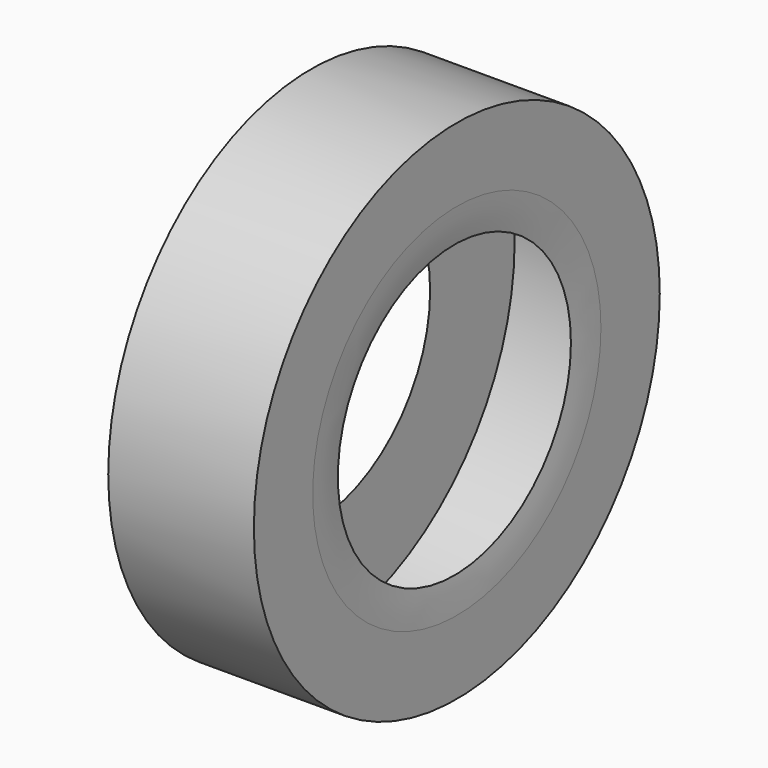
from build123d import *

# Parameters (mm, degrees)
F0_R     = 265.437423464
F0_R_2   = 152.4
F1_DEPTH = 152.4
F2_T     = -2.54


# Not quite as in the source:
# - a fillet or chamfer that OpenCascade refuses, or shapes differently, is made with other operations: its cross-section is extruded or revolved along the edge and cut away or added


with BuildPart() as f1:
    # F0 (on Right) → F1 (new body)
    with BuildSketch(Plane.YZ):
        Circle(F0_R)
        Circle(F0_R_2, mode=Mode.SUBTRACT)
    extrude(amount=F1_DEPTH)

    # F2
    f2_openings = [f1.faces().sort_by_distance(p)[0] for p in [
        (76.2, -152.4, 0),
    ]]
    offset(amount=F2_T, openings=f2_openings)

    # F3: fillet of radius 257.548302834 on 1 edges, made by hand

    # F3_s1 → F3_t2 (revolve, cut)
    with BuildSketch(Plane.XY):
        with BuildLine():
            ThreePointArc((152.4, 188.4817651785), (151.7642152496, 170.3962365824), (149.86, 152.4))
            Line((149.86, 152.4), (152.4, 152.4))
            Line((152.4, 152.4), (152.4, 188.4817651785))
        make_face()
    revolve(axis=Axis((152.4, 0, 0), (1, 0, 0)), mode=Mode.SUBTRACT)

    # F4: fillet of radius 331.1335322151 on 1 edges, made by hand

    # F4_s1 → F4_t2 (revolve, cut)
    with BuildSketch(Plane.XY):
        with BuildLine():
            ThreePointArc((0, 193.3353971967), (0.635610026, 172.828335342), (2.54, 152.4))
            Line((2.54, 152.4), (0, 152.4))
            Line((0, 152.4), (0, 193.3353971967))
        make_face()
    revolve(axis=Axis((0, 0, 0), (1, 0, 0)), mode=Mode.SUBTRACT)


solid = f1.part
